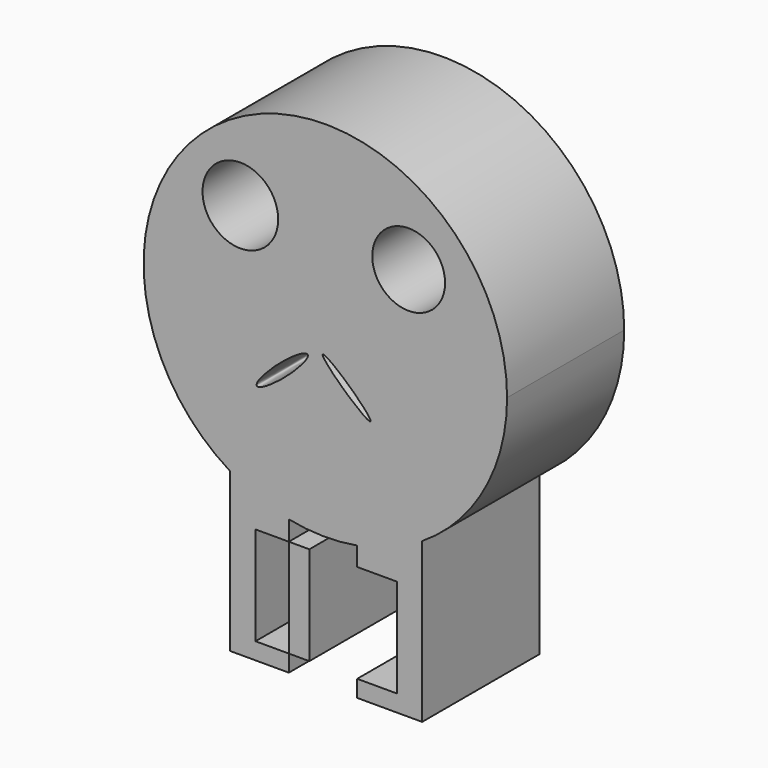
from build123d import *

# Parameters (mm, degrees)
F0_R     = 6.5620467743
F0_R_2   = 6.3170798388
F1_DEPTH = 25.4
F0_W     = 3.561691356
F0_H     = 17.082426697


with BuildPart() as f1:
    # F0 (on Front) → F1 (new body)
    with BuildSketch(Plane.XZ):
        with BuildLine():
            ThreePointArc((16.7904216796, 7.624526058), (27.5994929278, 19.0679390286), (31.5290121932, 34.3108586967))
            ThreePointArc((31.5290121932, 34.3108586967), (-15.3926210832, 61.8271416229), (-16.4995033487, 7.443685434))
            ThreePointArc((-16.4995033487, 7.443685434), (-11.5930935282, 4.9905791563), (-6.33576277, 3.4249926735))
            ThreePointArc((-6.33576277, 3.4249926735), (-0.4136566849, 2.7845601821), (5.5232139843, 3.2693909936))
            ThreePointArc((5.5232139843, 3.2693909936), (11.3673384965, 4.9023186889), (16.7904216796, 7.624526058))
        make_face()
        with BuildLine():
            add(Edge.make_bspline(
                [(-11.8729695678, 22.0014918596), (-10.7395709721, 20.6969963529), (-4.7141583751, 27.0767382417), (1.3112542219, 33.4564801306), (-5.8475569707, 28.3812337484), (-13.0063681634, 23.3059873662), (-11.8729695678, 22.0014918596)],
                knots=[0, 0, 0, 2.0943951024, 2.0943951024, 4.1887902048, 4.1887902048, 6.2831853072, 6.2831853072, 6.2831853072], degree=2, weights=[1, 0.5, 1, 0.5, 1, 0.5, 1]))
        make_face(mode=Mode.SUBTRACT)
        with Locations((-14.7463688627, 48.6192144454)):
            Circle(F0_R, mode=Mode.SUBTRACT)
        with BuildLine():
            add(Edge.make_bspline(
                [(7.8193116933, 22.9761805385), (8.5607238133, 23.7872275817), (1.9946380994, 29.0451604554), (-4.5714476146, 34.3030933291), (1.2532259794, 28.2341134122), (7.0778995733, 22.1651334954), (7.8193116933, 22.9761805385)],
                knots=[0, 0, 0, 2.0943951024, 2.0943951024, 4.1887902048, 4.1887902048, 6.2831853072, 6.2831853072, 6.2831853072], degree=2, weights=[1, 0.5, 1, 0.5, 1, 0.5, 1]))
        make_face(mode=Mode.SUBTRACT)
        with Locations((14.454362914, 48.3272075653)):
            Circle(F0_R_2, mode=Mode.SUBTRACT)
        with BuildLine():
            ThreePointArc((-6.33576277, 3.4249926735), (-11.5930935282, 4.9905791563), (-16.4995033487, 7.443685434))
            Line((-16.4995033487, 7.443685434), (-16.4995033487, -20.0025065972))
            Line((-16.4995033487, -20.0025065972), (-6.33576277, -20.0025065972))
            Line((-6.33576277, -20.0025065972), (-6.33576277, -17.082426697))
            Line((-6.33576277, -17.082426697), (-12.1183022857, -17.082426697))
            Line((-12.1183022857, -17.082426697), (-12.1183022857, 0))
            Line((-12.1183022857, 0), (-6.33576277, 0))
            Line((-6.33576277, 0), (-6.33576277, 3.4249926735))
        make_face()
        with BuildLine():
            Line((16.7904216796, -20.0025065972), (16.7904216796, 7.624526058))
            ThreePointArc((16.7904216796, 7.624526058), (11.3673384965, 4.9023186889), (5.5232139843, 3.2693909936))
            Line((5.5232139843, 3.2693909936), (5.5232139843, 0))
            Line((5.5232139843, 0), (12.4103091657, 0))
            Line((12.4103091657, 0), (12.4103091657, -17.082426697))
            Line((12.4103091657, -17.082426697), (5.5232139843, -17.082426697))
            Line((5.5232139843, -17.082426697), (5.5232139843, -20.0025065972))
            Line((5.5232139843, -20.0025065972), (16.7904216796, -20.0025065972))
        make_face()
    extrude(amount=F1_DEPTH)


with BuildPart() as f1b:
    # F0 (on Front) → F1, piece 2 (new body)
    with BuildSketch(Plane.XZ):
        with Locations((-4.554917092, -8.5412133485)):
            Rectangle(F0_W, F0_H)
    extrude(amount=F1_DEPTH)


solid = Compound([f1.part, f1b.part])
